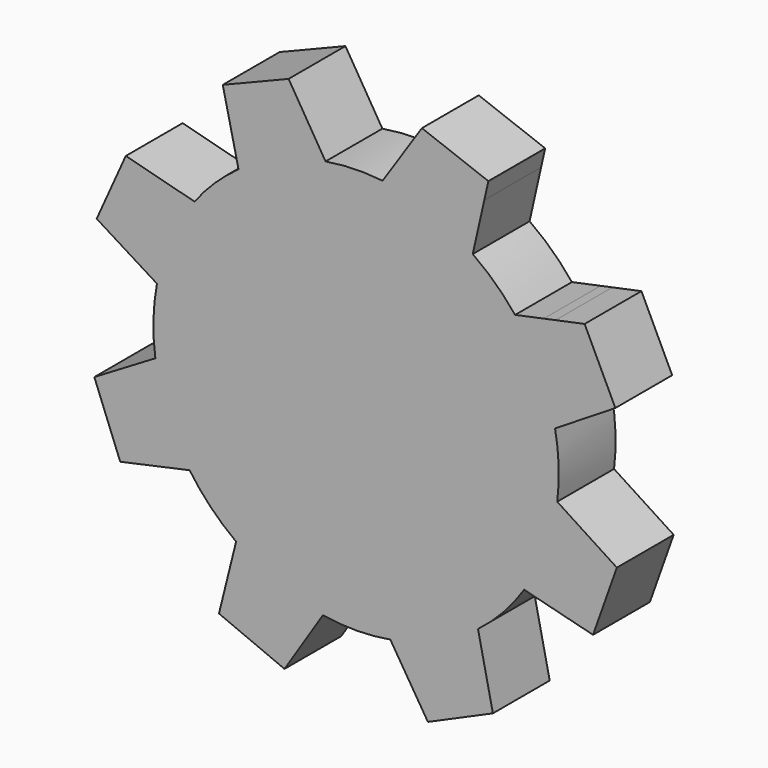
from build123d import *

# Parameters (mm, degrees)
F0_R     = 10.5352835121
F1_DEPTH = 10
F2_R     = 10.5352835121
F4_DEPTH = 10


with BuildPart() as f1:
    # F0 (on Front) → F1 (new body)
    with BuildSketch(Plane.XZ):
        with BuildLine():
            ThreePointArc((27.7799711237, -2.671018116), (28.1744534053, 0.0443174404), (28.3063539053, 2.7849862844))
            ThreePointArc((28.3063539053, 2.7849862844), (28.0187327637, 6.8265473039), (27.1616666974, 10.7866456806))
            ThreePointArc((27.1616666974, 10.7866456806), (25.7257105116, 14.6441244213), (23.7497903046, 18.2549209731))
            ThreePointArc((23.7497903046, 18.2549209731), (19.361792777, 23.5343393933), (13.840033917, 27.6131823971))
            ThreePointArc((13.840033917, 27.6131823971), (10.2093532061, 29.3452118388), (6.3712126192, 30.5495561611))
            ThreePointArc((6.3712126192, 30.5495561611), (-0.2384881302, 31.3241628205), (-6.8478808449, 30.5469322125))
            ThreePointArc((-6.8478808449, 30.5469322125), (-10.969919952, 29.2273648204), (-14.8450148239, 27.2996448624))
            ThreePointArc((-14.8450148239, 27.2996448624), (-20.0530528407, 23.3189368581), (-24.2154366907, 18.2549209731))
            ThreePointArc((-24.2154366907, 18.2549209731), (-26.4192319908, 14.132083875), (-27.9203856002, 9.7047780009))
            ThreePointArc((-27.9203856002, 9.7047780009), (-28.7702301145, 3.1028473381), (-28.0676480896, -3.5163748724))
            ThreePointArc((-28.0676480896, -3.5163748724), (-26.6541111331, -8.0039049024), (-24.5224980596, -12.1982151202))
            ThreePointArc((-24.5224980596, -12.1982151202), (-20.3786644673, -17.4296051981), (-15.133187526, -21.555592431))
            ThreePointArc((-15.133187526, -21.555592431), (-10.8750457734, -23.6957185401), (-6.3201455519, -25.0974299658))
            ThreePointArc((-6.3201455519, -25.0974299658), (0.4193178956, -25.7467388904), (7.122076621, -24.7901851235))
            ThreePointArc((7.122076621, -24.7901851235), (11.5833738131, -23.1931221487), (15.7189210631, -20.8798924315))
            ThreePointArc((15.7189210631, -20.8798924315), (20.7808637814, -16.5258808424), (24.6926258312, -11.1148921464))
            ThreePointArc((24.6926258312, -11.1148921464), (26.5708921122, -7.0152930628), (27.7799711237, -2.671018116))
        make_face()
        with Locations((-0.2328231931, 2.7849862844)):
            Circle(F0_R, mode=Mode.SUBTRACT)
        with BuildLine():
            ThreePointArc((-24.2154366907, 18.2549209731), (-20.0530528407, 23.3189368581), (-14.8450148239, 27.2996448624))
            Line((-14.8450148239, 27.2996448624), (-22.8760878199, 33.2579891401))
            Line((-22.8760878199, 33.2579891401), (-30.0983452841, 26.3414150516))
            Line((-30.0983452841, 26.3414150516), (-24.2154366907, 18.2549209731))
        make_face()
        with BuildLine():
            ThreePointArc((-28.0676480896, -3.5163748724), (-28.7702301145, 3.1028473381), (-27.9203856002, 9.7047780009))
            Line((-27.9203856002, 9.7047780009), (-37.8038170807, 8.1823515919))
            Line((-37.8038170807, 8.1823515919), (-37.9221875331, -1.8169478053))
            Line((-37.9221875331, -1.8169478053), (-28.0676480896, -3.5163748724))
        make_face()
        with BuildLine():
            Line((-23.298226533, -27.3289916042), (-15.133187526, -21.555592431))
            ThreePointArc((-15.133187526, -21.555592431), (-20.3786644673, -17.4296051981), (-24.5224980596, -12.1982151202))
            Line((-24.5224980596, -12.1982151202), (-30.3999287678, -20.2886915134))
            Line((-30.3999287678, -20.2886915134), (-23.298226533, -27.3289916042))
        make_face()
        with BuildLine():
            Line((5.3968944368, -34.640248394), (7.122076621, -24.7901851235))
            ThreePointArc((7.122076621, -24.7901851235), (0.4193178956, -25.7467388904), (-6.3201455519, -25.0974299658))
            Line((-6.3201455519, -25.0974299658), (-4.5983661602, -34.9480886101))
            Line((-4.5983661602, -34.9480886101), (5.3968944368, -34.640248394))
        make_face()
        with BuildLine():
            Line((30.4305433725, -19.3049044961), (24.6926258312, -11.1148921464))
            ThreePointArc((24.6926258312, -11.1148921464), (20.7808637814, -16.5258808424), (15.7189210631, -20.8798924315))
            Line((15.7189210631, -20.8798924315), (23.7909685899, -26.7826078003))
            Line((23.7909685899, -26.7826078003), (30.4305433725, -19.3049044961))
        make_face()
        with BuildLine():
            ThreePointArc((27.1616666974, 10.7866456806), (28.0187327637, 6.8265473039), (28.3063539053, 2.7849862844))
            ThreePointArc((28.3063539053, 2.7849862844), (28.1744534053, 0.0443174404), (27.7799711237, -2.671018116))
            Line((27.7799711237, -2.671018116), (37.6319898333, -0.9570381434))
            Line((37.6319898333, -0.9570381434), (37.004966841, 9.0232846052))
            Line((37.004966841, 9.0232846052), (27.1616666974, 10.7866456806))
        make_face()
        with BuildLine():
            ThreePointArc((13.840033917, 27.6131823971), (19.361792777, 23.5343393933), (23.7497903046, 18.2549209731))
            Line((23.7497903046, 18.2549209731), (29.4473420196, 26.4730658036))
            Line((29.4473420196, 26.4730658036), (22.097377097, 33.2537748843))
            Line((22.097377097, 33.2537748843), (13.840033917, 27.6131823971))
        make_face()
        with BuildLine():
            ThreePointArc((-6.8478808449, 30.5469322125), (-0.2384881302, 31.3241628205), (6.3712126192, 30.5495561611))
            Line((6.3712126192, 30.5495561611), (4.7536209633, 40.4178588133))
            Line((4.7536209633, 40.4178588133), (-5.2463790367, 40.4178588133))
            Line((-5.2463790367, 40.4178588133), (-6.8478808449, 30.5469322125))
        make_face()
    extrude(amount=F1_DEPTH)


with BuildPart() as f4:
    # F2 (on face) → F4 (new body)
    with BuildSketch(Plane.XZ.offset(10)):
        with BuildLine():
            Line((6.0436061547, -23.2930321543), (3.9465958394, -13.5153766205))
            ThreePointArc((3.9465958394, -13.5153766205), (7.4913970999, -10.2975314551), (10.4484246026, -6.5324110277))
            Line((10.4484246026, -6.5324110277), (20.145561814, -8.9748544564))
            Line((20.145561814, -8.9748544564), (23.4940421304, 0.4478669961))
            Line((23.4940421304, 0.4478669961), (15.1021918552, 5.8863271605))
            ThreePointArc((15.1021918552, 5.8863271605), (15.3048791393, 10.3911595364), (14.795466022, 14.8716835175))
            Line((14.795466022, 14.8716835175), (23.2844256021, 20.1572833176))
            Line((23.2844256021, 20.1572833176), (18.9582119637, 29.1730403882))
            Line((18.9582119637, 29.1730403882), (14.8616590906, 28.3110547216))
            Line((14.8616590906, 28.3110547216), (13.840033917, 27.6131823971))
            ThreePointArc((13.840033917, 27.6131823971), (13.5236804737, 27.7898505375), (13.2051095461, 27.9624880101))
            Line((13.2051095461, 27.9624880101), (9.1724991444, 27.1139569468))
            ThreePointArc((9.1724991444, 27.1139569468), (6.3915510384, 30.1271942866), (3.2074944908, 32.7108071709))
            Line((3.2074944908, 32.7108071709), (4.8336037454, 39.9299147155))
            Line((4.8336037454, 39.9299147155), (4.7536209633, 40.4178588133))
            Line((4.7536209633, 40.4178588133), (-5.2463790367, 40.4178588133))
            Line((-5.2463790367, 40.4178588133), (-6.8478808449, 30.5469322125))
            ThreePointArc((-6.8478808449, 30.5469322125), (-10.969919952, 29.2273648204), (-14.8450148239, 27.2996448624))
            Line((-14.8450148239, 27.2996448624), (-22.8760878199, 33.2579891401))
            Line((-22.8760878199, 33.2579891401), (-30.0983452841, 26.3414150516))
            Line((-30.0983452841, 26.3414150516), (-24.2154366907, 18.2549209731))
            ThreePointArc((-24.2154366907, 18.2549209731), (-26.4192319908, 14.132083875), (-27.9203856002, 9.7047780009))
            Line((-27.9203856002, 9.7047780009), (-37.8038170807, 8.1823515919))
            Line((-37.8038170807, 8.1823515919), (-37.9221875331, -1.8169478053))
            Line((-37.9221875331, -1.8169478053), (-28.0676480896, -3.5163748724))
            ThreePointArc((-28.0676480896, -3.5163748724), (-26.6541111331, -8.0039049024), (-24.5224980596, -12.1982151202))
            Line((-24.5224980596, -12.1982151202), (-30.3999287678, -20.2886915134))
            Line((-30.3999287678, -20.2886915134), (-23.298226533, -27.3289916042))
            Line((-23.298226533, -27.3289916042), (-17.896228959, -18.9136233882))
            ThreePointArc((-17.896228959, -18.9136233882), (-13.1442498661, -19.2768415054), (-8.3980860704, -18.8442193547))
            Line((-8.3980860704, -18.8442193547), (-3.10576712, -27.3289916042))
            Line((-3.10576712, -27.3289916042), (6.0436061547, -23.2930321543))
        make_face()
        with Locations((-0.2328231931, 2.7849862844)):
            Circle(F2_R, mode=Mode.SUBTRACT)
        with BuildLine():
            Line((-32.5227899129, -23.4679774305), (-23.298226533, -27.3289916042))
            Line((-23.298226533, -27.3289916042), (-30.3999287678, -20.2886915134))
            Line((-30.3999287678, -20.2886915134), (-24.5224980596, -12.1982151202))
            ThreePointArc((-24.5224980596, -12.1982151202), (-26.6541111331, -8.0039049024), (-28.0676480896, -3.5163748724))
            Line((-28.0676480896, -3.5163748724), (-37.9221875331, -1.8169478053))
            Line((-37.9221875331, -1.8169478053), (-37.8038170807, 8.1823515919))
            Line((-37.8038170807, 8.1823515919), (-27.9203856002, 9.7047780009))
            ThreePointArc((-27.9203856002, 9.7047780009), (-26.4192319908, 14.132083875), (-24.2154366907, 18.2549209731))
            Line((-24.2154366907, 18.2549209731), (-30.0983452841, 26.3414150516))
            Line((-30.0983452841, 26.3414150516), (-22.8760878199, 33.2579891401))
            Line((-22.8760878199, 33.2579891401), (-14.8450148239, 27.2996448624))
            ThreePointArc((-14.8450148239, 27.2996448624), (-10.969919952, 29.2273648204), (-6.8478808449, 30.5469322125))
            Line((-6.8478808449, 30.5469322125), (-5.2463790367, 40.4178588133))
            Line((-5.2463790367, 40.4178588133), (4.7536209633, 40.4178588133))
            Line((4.7536209633, 40.4178588133), (4.8336037454, 39.9299147155))
            Line((4.8336037454, 39.9299147155), (5.3773912439, 42.3440578129))
            Line((5.3773912439, 42.3440578129), (5.4049445449, 42.4663806169))
            Line((5.4049445449, 42.4663806169), (-3.952331747, 45.9936147169))
            Line((-3.952331747, 45.9936147169), (-9.4897229207, 37.6667125925))
            ThreePointArc((-9.4897229207, 37.6667125925), (-13.5099465153, 37.8436589686), (-17.5150931781, 37.4533924182))
            Line((-17.5150931781, 37.4533924182), (-22.7174583218, 45.9936147169))
            Line((-22.7174583218, 45.9936147169), (-31.9867384026, 42.2412225755))
            Line((-31.9867384026, 42.2412225755), (-29.767256543, 32.4906379635))
            ThreePointArc((-29.767256543, 32.4906379635), (-33.0929366105, 29.720743274), (-35.9615144592, 26.4797980987))
            Line((-35.9615144592, 26.4797980987), (-45.6415453785, 28.9891807718))
            Line((-45.6415453785, 28.9891807718), (-49.7406882781, 19.867940314))
            Line((-49.7406882781, 19.867940314), (-41.2532858507, 14.5798404628))
            ThreePointArc((-41.2532858507, 14.5798404628), (-41.7489952856, 9.9313168673), (-41.4791578337, 5.2642313516))
            Line((-41.4791578337, 5.2642313516), (-50.0691131996, 0.1444006111))
            Line((-50.0691131996, 0.1444006111), (-46.4267048395, -9.168647297))
            Line((-46.4267048395, -9.168647297), (-36.6545645454, -7.0460842067))
            ThreePointArc((-36.6545645454, -7.0460842067), (-33.660420308, -10.6752869818), (-30.1106987778, -13.7632457827))
            Line((-30.1106987778, -13.7632457827), (-32.5227899129, -23.4679774305))
        make_face()
        with BuildLine():
            Line((13.840033917, 27.6131823971), (14.8616590906, 28.3110547216))
            Line((14.8616590906, 28.3110547216), (13.2051095461, 27.9624880101))
            ThreePointArc((13.2051095461, 27.9624880101), (13.5236804737, 27.7898505375), (13.840033917, 27.6131823971))
        make_face()
        with Locations((-0.2328231931, 2.7849862844)):
            Circle(F2_R)
    extrude(amount=F4_DEPTH)


solid = f4.part
